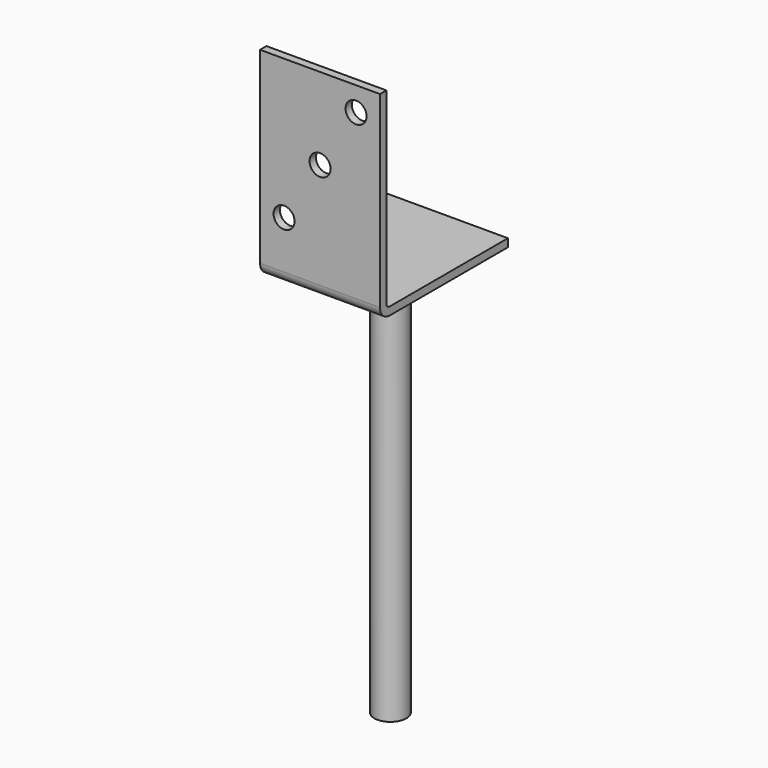
from build123d import *

# Parameters (mm, degrees)
F1_DEPTH = 30
F2_R     = 8
F3_DEPTH = 200
F5_R     = 2
F6_R     = 6
F4_R     = 5.25
F7_DEPTH = 25


# Not quite as in the source:
# - a feature names something its author has since deleted; it is built from what else it names


with BuildPart() as f1:
    # F0 (on Right) → F1 (new body, symmetric)
    with BuildSketch(Plane.YZ):
        Polygon((36, -50), (-40, -50), (-40, 46), (-44, 46), (-44, -54), (36, -54), align=None)
    extrude(amount=F1_DEPTH, both=True)

    # F2 (on face) → F3 (join)
    with BuildSketch(Plane(origin=(0, 0, -54), x_dir=(1, 0, 0), z_dir=(0, 0, -1))):
        Circle(F2_R)
    extrude(amount=F3_DEPTH)

    # F5
    f5_edges = [f1.edges().sort_by_distance(p)[0] for p in [
        (0, -40, -50),
    ]]
    fillet(f5_edges, radius=F5_R)

    # F6
    f6_edges = [f1.edges().sort_by_distance(p)[0] for p in [
        (0, -44, -54),
    ]]
    fillet(f6_edges, radius=F6_R)

    # F4 (on face) → F7 (cut)
    with BuildSketch(Plane.XZ.offset(44)):
        with Locations((18, 34)):
            Circle(F4_R)
        with Locations((0, 5)):
            Circle(F4_R)
        with Locations((-18, -24)):
            Circle(F4_R)
    extrude(amount=-F7_DEPTH, mode=Mode.SUBTRACT)


solid = f1.part
